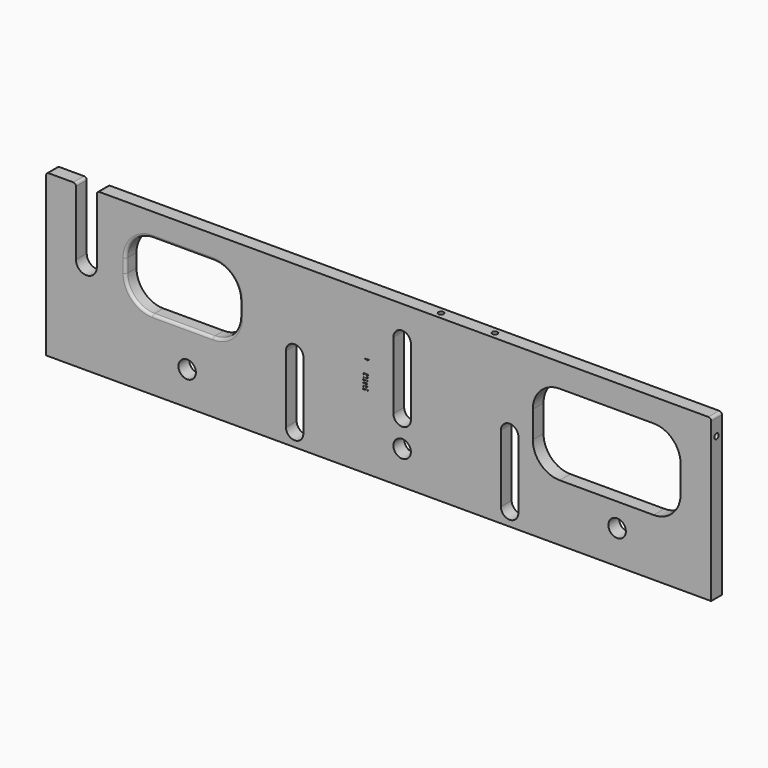
from build123d import *

# Parameters (mm, degrees)
F0_R           = 6.5
F1_DEPTH       = 5
F2_R           = 2
F3_DEPTH       = 10
F4_R           = 2
F5_R           = 2
F7_DEPTH       = 10
F6_R           = 2
F8_DEPTH       = 10
F9_W           = 5
F9_H           = 0.0002
F9_W_2         = 2.5
F9_H_2         = 0.0002000006
F9_TEXT_SIZE   = 1.3888888887
F9_TEXT_SIZE_2 = 1.4578467426
F9_TEXT_SIZE_3 = 1.2903071769
F9_TEXT_SIZE_4 = 1.4170512758
F9_TEXT_SIZE_5 = 1.3888888891
F9_TEXT_SIZE_6 = 1.3957622474
F9_TEXT_SIZE_7 = 1.3792238209
F10_DEPTH      = 0.5
F11_R          = 2


# Not quite as in the source:
# - Text() gives the source's letters only with a copy of the font that has no kerning and outlines rounded to 1/6400 em; it was checked with that copy


with BuildPart() as f1:
    # F0 (on Front) → F1 (new body, symmetric)
    with BuildSketch(Plane.XZ):
        with BuildLine():
            Line((-247.5, 60), (-247.5, -60))
            Line((-247.5, -60), (247.5, -60))
            Line((247.5, -60), (247.5, 60))
            Line((247.5, 60), (-209.75, 60))
            Line((-209.75, 60), (-209.75, 10))
            ThreePointArc((-209.75, 10), (-217.5, 2.25), (-225.25, 10))
            Line((-225.25, 10), (-225.25, 60))
            Line((-225.25, 60), (-247.5, 60))
        make_face()
        with Locations((-142.5, -35)):
            Circle(F0_R, mode=Mode.SUBTRACT)
        with BuildLine():
            ThreePointArc((-56, -49), (-62.5, -55.5), (-69, -49))
            Line((-69, -49), (-69, 1))
            ThreePointArc((-69, 1), (-62.5, 7.5), (-56, 1))
            Line((-56, 1), (-56, -49))
        make_face(mode=Mode.SUBTRACT)
        with Locations((17.5, -35)):
            Circle(F0_R, mode=Mode.SUBTRACT)
        with Locations((177.5, -35)):
            Circle(F0_R, mode=Mode.SUBTRACT)
        with BuildLine():
            ThreePointArc((104, -49), (97.5, -55.5), (91, -49))
            Line((91, -49), (91, 1))
            ThreePointArc((91, 1), (97.5, 7.5), (104, 1))
            Line((104, 1), (104, -49))
        make_face(mode=Mode.SUBTRACT)
        with BuildLine():
            ThreePointArc((-188.2200682163, 22.5), (-182.3622038401, 36.6421356237), (-168.2200682163, 42.5))
            Line((-168.2200682163, 42.5), (-123.2200682163, 42.5))
            ThreePointArc((-123.2200682163, 42.5), (-109.0779325926, 36.6421356237), (-103.2200682163, 22.5))
            Line((-103.2200682163, 22.5), (-103.2200682163, 12.5))
            ThreePointArc((-103.2200682163, 12.5), (-109.0779325926, -1.6421356237), (-123.2200682163, -7.5))
            Line((-123.2200682163, -7.5), (-168.2200682163, -7.5))
            ThreePointArc((-168.2200682163, -7.5), (-182.3622038401, -1.6421356237), (-188.2200682163, 12.5))
            Line((-188.2200682163, 12.5), (-188.2200682163, 22.5))
        make_face(mode=Mode.SUBTRACT)
        with BuildLine():
            ThreePointArc((24, -14), (17.5, -20.5), (11, -14))
            Line((11, -14), (11, 36))
            ThreePointArc((11, 36), (17.5, 42.5), (24, 36))
            Line((24, 36), (24, -14))
        make_face(mode=Mode.SUBTRACT)
        with BuildLine():
            ThreePointArc((114.7344782948, 22.5), (120.5923426711, 36.6421356237), (134.7344782948, 42.5))
            Line((134.7344782948, 42.5), (204.7344782948, 42.5))
            ThreePointArc((204.7344782948, 42.5), (218.8766139186, 36.6421356237), (224.7344782948, 22.5))
            Line((224.7344782948, 22.5), (224.7344782948, 2.5))
            ThreePointArc((224.7344782948, 2.5), (218.8766139186, -11.6421356237), (204.7344782948, -17.5))
            Line((204.7344782948, -17.5), (134.7344782948, -17.5))
            ThreePointArc((134.7344782948, -17.5), (120.5923426711, -11.6421356237), (114.7344782948, 2.5))
            Line((114.7344782948, 2.5), (114.7344782948, 22.5))
        make_face(mode=Mode.SUBTRACT)
    extrude(amount=F1_DEPTH, both=True)

    # F2 (on face) → F3 (cut)
    with BuildSketch(Plane.XY.offset(60)):
        with Locations((42.5, 0)):
            Circle(F2_R)
        with Locations((82.5, 0)):
            Circle(F2_R)
    extrude(amount=-F3_DEPTH, mode=Mode.SUBTRACT)

    # F4
    f4_edges = [f1.edges().sort_by_distance(p)[0] for p in [
        (-225.25, 0, 60),
        (-247.5, 0, 60),
        (-209.75, 0, 60),
        (247.5, 0, 60),
    ]]
    fillet(f4_edges, radius=F4_R)

    # F5 (on face) → F7 (cut)
    with BuildSketch(Plane(origin=(-247.5, 0, 0), x_dir=(0, -1, 0), z_dir=(-1, 0, 0))):
        with Locations((0, 46)):
            Circle(F5_R)
    extrude(amount=-F7_DEPTH, mode=Mode.SUBTRACT)

    # F6 (on face) → F8 (cut)
    with BuildSketch(Plane.YZ.offset(247.5)):
        with Locations((0, 46)):
            Circle(F6_R)
    extrude(amount=-F8_DEPTH, mode=Mode.SUBTRACT)

    # F9 (on face) → F10 (cut)
    with BuildSketch(Plane.XZ.offset(5)):
        with Locations((-14.5, -5.9959875856)):
            Rectangle(F9_W, F9_H)
        with Locations((-13.25, -5.4959662829)):
            Rectangle(F9_W_2, F9_H)
        with Locations((-14.5, -4.9959449804)):
            Rectangle(F9_W, F9_H)
        with Locations((-14.5, -3.9959449804)):
            Rectangle(F9_W, F9_H)
        with Locations((-13.25, -4.4959662831)):
            Rectangle(F9_W_2, F9_H)
        with Locations((-13.25, -3.4959662829)):
            Rectangle(F9_W_2, F9_H)
        with Locations((-14.5, -1.9959875849)):
            Rectangle(F9_W, F9_H)
        with Locations((-14.5, -0.9959449797)):
            Rectangle(F9_W, F9_H)
        with Locations((-13.25, -1.4959662824)):
            Rectangle(F9_W_2, F9_H)
        with Locations((-13.25, -2.4959662822)):
            Rectangle(F9_W_2, F9_H)
        with Locations((-14.5, -2.9959875849)):
            Rectangle(F9_W, F9_H)
        with Locations((-13.25, -0.4959662822)):
            Rectangle(F9_W_2, F9_H)
        with Locations((-13.25, 1.5040337178)):
            Rectangle(F9_W_2, F9_H)
        with Locations((-14.5, 0.0040124153)):
            Rectangle(F9_W, F9_H)
        with Locations((-14.5, 4.004012416)):
            Rectangle(F9_W, F9_H)
        with Locations((-14.5, 5.0040550211)):
            Rectangle(F9_W, F9_H)
        with Locations((-14.5, 1.0040550204)):
            Rectangle(F9_W, F9_H)
        with Locations((-13.25, 2.5040337182)):
            Rectangle(F9_W_2, F9_H_2)
        with Locations((-13.25, 3.5040337187)):
            Rectangle(F9_W_2, F9_H)
        with Locations((-14.5, 2.0040550204)):
            Rectangle(F9_W, F9_H)
        with Locations((-14.5, 3.004012416)):
            Rectangle(F9_W, F9_H)
        with Locations((-13.25, 0.5040337179)):
            Rectangle(F9_W_2, F9_H)
        with Locations((-13.25, 4.5040337185)):
            Rectangle(F9_W_2, F9_H)
        with Locations((-13.25, 5.5040337187)):
            Rectangle(F9_W_2, F9_H)
        with Locations((-13.25, 6.5040337172)):
            Rectangle(F9_W_2, F9_H)
        with Locations((-14.5, 7.0040550197)):
            Rectangle(F9_W, F9_H)
        with Locations((-13.25, 7.5040337171)):
            Rectangle(F9_W_2, F9_H)
        with Locations((-14.5, 16.0040124162)):
            Rectangle(F9_W, F9_H)
        with Locations((-14.5, 9.0040124153)):
            Rectangle(F9_W, F9_H)
        with Locations((-13.25, 11.5040337179)):
            Rectangle(F9_W_2, F9_H)
        with Locations((-14.5, 14.0040550206)):
            Rectangle(F9_W, F9_H)
        with Locations((-14.5, 10.0040124153)):
            Rectangle(F9_W, F9_H)
        with Locations((-13.25, 15.5040337188)):
            Rectangle(F9_W_2, F9_H)
        with Locations((-14.5, 11.0040550204)):
            Rectangle(F9_W, F9_H)
        with Locations((-14.5, 6.0040124146)):
            Rectangle(F9_W, F9_H)
        with Locations((-13.25, 8.5040337172)):
            Rectangle(F9_W_2, F9_H)
        with Locations((-13.25, 10.5040337178)):
            Rectangle(F9_W_2, F9_H)
        with Locations((-14.5, 15.0040124162)):
            Rectangle(F9_W, F9_H)
        with Locations((-14.5, 8.0040550197)):
            Rectangle(F9_W, F9_H)
        with Locations((-13.25, 14.5040337184)):
            Rectangle(F9_W_2, F9_H_2)
        with Locations((-13.25, 13.5040337179)):
            Rectangle(F9_W_2, F9_H)
        with Locations((-14.5, 12.0040124154)):
            Rectangle(F9_W, F9_H)
        with Locations((-13.25, 16.5040337187)):
            Rectangle(F9_W_2, F9_H)
        with Locations((-13.25, 12.5040337181)):
            Rectangle(F9_W_2, F9_H)
        with Locations((-14.5, 17.0040550213)):
            Rectangle(F9_W, F9_H)
        with Locations((-14.5, 13.0040550206)):
            Rectangle(F9_W, F9_H)
        with Locations((-13.25, 9.5040337179)):
            Rectangle(F9_W_2, F9_H)
        with Locations((-11.6391059028, -5.4958662829)):
            Text('0 mm', F9_TEXT_SIZE, font='Open Sans', text_align=(TextAlign.LEFT, TextAlign.BOTTOM))
        with Locations((-11.6211876355, -3.5455159369)):
            Text('2 mm', F9_TEXT_SIZE_2, font='Open Sans', text_align=(TextAlign.LEFT, TextAlign.BOTTOM))
        with Locations((-11.6647217445, -1.4248874496)):
            Text('4 mm', F9_TEXT_SIZE_3, font='Open Sans', text_align=(TextAlign.LEFT, TextAlign.BOTTOM))
        with Locations((-11.6317880825, 0.4838567992)):
            Text('6 mm', F9_TEXT_SIZE_4, font='Open Sans', text_align=(TextAlign.LEFT, TextAlign.BOTTOM))
        with Locations((-11.4928166513, 2.5041337185)):
            Text('8 mm', F9_TEXT_SIZE_5, font='Open Sans', text_align=(TextAlign.LEFT, TextAlign.BOTTOM))
        with Locations((-11.4910306521, 4.4991849005)):
            Text('10 mm', F9_TEXT_SIZE_6, font='Open Sans', text_align=(TextAlign.LEFT, TextAlign.BOTTOM))
        with Locations((-11.4425947117, 14.5110925678)):
            Text('20 mm', F9_TEXT_SIZE_7, font='Open Sans', text_align=(TextAlign.LEFT, TextAlign.BOTTOM))
    extrude(amount=-F10_DEPTH, mode=Mode.SUBTRACT)

    # F11
    f11_edges = [f1.edges().sort_by_distance(p)[0] for p in [
        (-145.720068, -5, -7.5),
        (-182.362204, -5, 36.642136),
        (-182.362204, -5, -1.642136),
        (-188.220068, -5, 17.5),
        (-145.720068, -5, 42.5),
        (-109.077933, -5, 36.642136),
        (-103.220068, -5, 17.5),
        (-109.077933, -5, -1.642136),
    ]]
    fillet(f11_edges, radius=F11_R)


solid = f1.part
